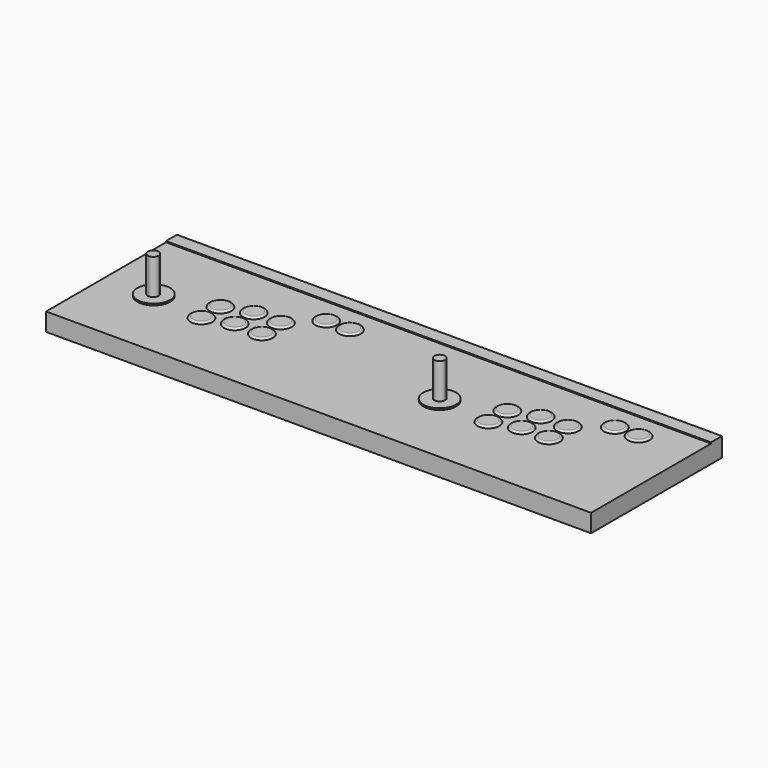
from build123d import *

# Parameters (mm, degrees)
F0_W     = 1000
F0_H     = 35
F1_DEPTH = 300
F2_W     = 1000
F2_H     = 275
F3_DEPTH = 2
F4_R     = 30
F4_R_2   = 20
F5_DEPTH = 3
F8_DEPTH = 65


# Not quite as in the source:
# - a fillet or chamfer that OpenCascade refuses, or shapes differently, is made with other operations: its cross-section is extruded or revolved along the edge and cut away or added


with BuildPart() as f1:
    # F0 (on Front) → F1 (new body)
    with BuildSketch(Plane.XZ):
        with Locations((415.1359161552, 9.4094127417)):
            Rectangle(F0_W, F0_H)
    extrude(amount=F1_DEPTH)

    # F2 (on face) → F3 (cut)
    with BuildSketch(Plane.XY.offset(26.9094127417)):
        with Locations((415.1359161552, -162.5)):
            Rectangle(F2_W, F2_H)
    extrude(amount=-F3_DEPTH, mode=Mode.SUBTRACT)

    # F4 (on face) → F5 (join)
    with BuildSketch(Plane.XY.offset(24.9094127417)):
        with Locations((5.3150048805, -165.6954972839)):
            Circle(F4_R)
        with Locations((101.5675663948, -176.7151132226)):
            Circle(F4_R_2)
        with Locations((101.5675638381, -133.2076661438)):
            Circle(F4_R_2)
        with Locations((150.2870444718, -117.7002512067)):
            Circle(F4_R_2)
        with Locations((200.0602781773, -161.2076982856)):
            Circle(F4_R_2)
        with Locations((200.0602756206, -117.7002512067)):
            Circle(F4_R_2)
        with Locations((150.2870470285, -161.2076982856)):
            Circle(F4_R_2)
        with Locations((247.0354534834, -72.4265153941)):
            Circle(F4_R_2)
        with Locations((290.5429005623, -72.4265128374)):
            Circle(F4_R_2)
        with Locations((527.8573036194, -163.2558181882)):
            Circle(F4_R)
        with Locations((624.1627931595, -171.8313768506)):
            Circle(F4_R_2)
        with Locations((624.1627906028, -128.3239297718)):
            Circle(F4_R_2)
        with Locations((672.8822712365, -112.8165148347)):
            Circle(F4_R_2)
        with Locations((672.8822737932, -156.3239619136)):
            Circle(F4_R_2)
        with Locations((722.6555049419, -156.3239619136)):
            Circle(F4_R_2)
        with Locations((722.6555023852, -112.8165148347)):
            Circle(F4_R_2)
        with Locations((776.1480905264, -71.8160520729)):
            Circle(F4_R_2)
        with Locations((819.6555376053, -71.8160495162)):
            Circle(F4_R_2)
    extrude(amount=F5_DEPTH)

    # F6: fillet of radius 5 on 16 edges, made by hand

    # F6_s1 → F6_t2 (revolve, cut)
    with BuildSketch(Plane.XZ.offset(176.7151132226)):
        with BuildLine():
            ThreePointArc((121.5675663948, 24.9094127417), (119.7236034874, 27.0927128743), (116.9849906999, 27.9094127417))
            Line((116.9849906999, 27.9094127417), (121.5675663948, 27.9094127417))
            Line((121.5675663948, 27.9094127417), (121.5675663948, 24.9094127417))
        make_face()
    revolve(axis=Axis((101.5675663948, -176.7151132226, 27.9094127417), (0, 0, 1)), mode=Mode.SUBTRACT)

    # F6_s3 → F6_t4 (revolve, cut)
    with BuildSketch(Plane.XZ.offset(133.2076661438)):
        with BuildLine():
            ThreePointArc((121.5675638381, 24.9094127417), (119.7236009307, 27.0927128743), (116.9849881431, 27.9094127417))
            Line((116.9849881431, 27.9094127417), (121.5675638381, 27.9094127417))
            Line((121.5675638381, 27.9094127417), (121.5675638381, 24.9094127417))
        make_face()
    revolve(axis=Axis((101.5675638381, -133.2076661438, 27.9094127417), (0, 0, 1)), mode=Mode.SUBTRACT)

    # F6_s5 → F6_t6 (revolve, cut)
    with BuildSketch(Plane.XZ.offset(117.7002512067)):
        with BuildLine():
            ThreePointArc((170.2870444718, 24.9094127417), (168.4430815644, 27.0927128743), (165.7044687769, 27.9094127417))
            Line((165.7044687769, 27.9094127417), (170.2870444718, 27.9094127417))
            Line((170.2870444718, 27.9094127417), (170.2870444718, 24.9094127417))
        make_face()
    revolve(axis=Axis((150.2870444718, -117.7002512067, 27.9094127417), (0, 0, 1)), mode=Mode.SUBTRACT)

    # F6_s7 → F6_t8 (revolve, cut)
    with BuildSketch(Plane.XZ.offset(161.2076982856)):
        with BuildLine():
            ThreePointArc((170.2870470285, 24.9094127417), (168.4430841211, 27.0927128743), (165.7044713336, 27.9094127417))
            Line((165.7044713336, 27.9094127417), (170.2870470285, 27.9094127417))
            Line((170.2870470285, 27.9094127417), (170.2870470285, 24.9094127417))
        make_face()
    revolve(axis=Axis((150.2870470285, -161.2076982856, 27.9094127417), (0, 0, 1)), mode=Mode.SUBTRACT)

    # F6_s9 → F6_t10 (revolve, cut)
    with BuildSketch(Plane.XZ.offset(161.2076982856)):
        with BuildLine():
            ThreePointArc((220.0602781773, 24.9094127417), (218.2163152698, 27.0927128743), (215.4777024823, 27.9094127417))
            Line((215.4777024823, 27.9094127417), (220.0602781773, 27.9094127417))
            Line((220.0602781773, 27.9094127417), (220.0602781773, 24.9094127417))
        make_face()
    revolve(axis=Axis((200.0602781773, -161.2076982856, 27.9094127417), (0, 0, 1)), mode=Mode.SUBTRACT)

    # F6_s11 → F6_t12 (revolve, cut)
    with BuildSketch(Plane.XZ.offset(117.7002512067)):
        with BuildLine():
            ThreePointArc((220.0602756206, 24.9094127417), (218.2163127131, 27.0927128743), (215.4776999256, 27.9094127417))
            Line((215.4776999256, 27.9094127417), (220.0602756206, 27.9094127417))
            Line((220.0602756206, 27.9094127417), (220.0602756206, 24.9094127417))
        make_face()
    revolve(axis=Axis((200.0602756206, -117.7002512067, 27.9094127417), (0, 0, 1)), mode=Mode.SUBTRACT)

    # F6_s13 → F6_t14 (revolve, cut)
    with BuildSketch(Plane.XZ.offset(72.4265153941)):
        with BuildLine():
            ThreePointArc((267.0354534834, 24.9094127417), (265.191490576, 27.0927128743), (262.4528777885, 27.9094127417))
            Line((262.4528777885, 27.9094127417), (267.0354534834, 27.9094127417))
            Line((267.0354534834, 27.9094127417), (267.0354534834, 24.9094127417))
        make_face()
    revolve(axis=Axis((247.0354534834, -72.4265153941, 27.9094127417), (0, 0, 1)), mode=Mode.SUBTRACT)

    # F6_s15 → F6_t16 (revolve, cut)
    with BuildSketch(Plane.XZ.offset(72.4265128374)):
        with BuildLine():
            ThreePointArc((310.5429005623, 24.9094127417), (308.6989376549, 27.0927128743), (305.9603248673, 27.9094127417))
            Line((305.9603248673, 27.9094127417), (310.5429005623, 27.9094127417))
            Line((310.5429005623, 27.9094127417), (310.5429005623, 24.9094127417))
        make_face()
    revolve(axis=Axis((290.5429005623, -72.4265128374, 27.9094127417), (0, 0, 1)), mode=Mode.SUBTRACT)

    # F6_s17 → F6_t18 (revolve, cut)
    with BuildSketch(Plane.XZ.offset(71.8160495162)):
        with BuildLine():
            ThreePointArc((839.6555376053, 24.9094127417), (837.8115746979, 27.0927128743), (835.0729619103, 27.9094127417))
            Line((835.0729619103, 27.9094127417), (839.6555376053, 27.9094127417))
            Line((839.6555376053, 27.9094127417), (839.6555376053, 24.9094127417))
        make_face()
    revolve(axis=Axis((819.6555376053, -71.8160495162, 27.9094127417), (0, 0, 1)), mode=Mode.SUBTRACT)

    # F6_s19 → F6_t20 (revolve, cut)
    with BuildSketch(Plane.XZ.offset(71.8160520729)):
        with BuildLine():
            ThreePointArc((796.1480905264, 24.9094127417), (794.304127619, 27.0927128743), (791.5655148315, 27.9094127417))
            Line((791.5655148315, 27.9094127417), (796.1480905264, 27.9094127417))
            Line((796.1480905264, 27.9094127417), (796.1480905264, 24.9094127417))
        make_face()
    revolve(axis=Axis((776.1480905264, -71.8160520729, 27.9094127417), (0, 0, 1)), mode=Mode.SUBTRACT)

    # F6_s21 → F6_t22 (revolve, cut)
    with BuildSketch(Plane.XZ.offset(112.8165148347)):
        with BuildLine():
            ThreePointArc((742.6555023852, 24.9094127417), (740.8115394778, 27.0927128743), (738.0729266903, 27.9094127417))
            Line((738.0729266903, 27.9094127417), (742.6555023852, 27.9094127417))
            Line((742.6555023852, 27.9094127417), (742.6555023852, 24.9094127417))
        make_face()
    revolve(axis=Axis((722.6555023852, -112.8165148347, 27.9094127417), (0, 0, 1)), mode=Mode.SUBTRACT)

    # F6_s23 → F6_t24 (revolve, cut)
    with BuildSketch(Plane.XZ.offset(156.3239619136)):
        with BuildLine():
            ThreePointArc((742.6555049419, 24.9094127417), (740.8115420345, 27.0927128743), (738.072929247, 27.9094127417))
            Line((738.072929247, 27.9094127417), (742.6555049419, 27.9094127417))
            Line((742.6555049419, 27.9094127417), (742.6555049419, 24.9094127417))
        make_face()
    revolve(axis=Axis((722.6555049419, -156.3239619136, 27.9094127417), (0, 0, 1)), mode=Mode.SUBTRACT)

    # F6_s25 → F6_t26 (revolve, cut)
    with BuildSketch(Plane.XZ.offset(156.3239619136)):
        with BuildLine():
            ThreePointArc((692.8822737932, 24.9094127417), (691.0383108858, 27.0927128743), (688.2996980983, 27.9094127417))
            Line((688.2996980983, 27.9094127417), (692.8822737932, 27.9094127417))
            Line((692.8822737932, 27.9094127417), (692.8822737932, 24.9094127417))
        make_face()
    revolve(axis=Axis((672.8822737932, -156.3239619136, 27.9094127417), (0, 0, 1)), mode=Mode.SUBTRACT)

    # F6_s27 → F6_t28 (revolve, cut)
    with BuildSketch(Plane.XZ.offset(112.8165148347)):
        with BuildLine():
            ThreePointArc((692.8822712365, 24.9094127417), (691.0383083291, 27.0927128743), (688.2996955416, 27.9094127417))
            Line((688.2996955416, 27.9094127417), (692.8822712365, 27.9094127417))
            Line((692.8822712365, 27.9094127417), (692.8822712365, 24.9094127417))
        make_face()
    revolve(axis=Axis((672.8822712365, -112.8165148347, 27.9094127417), (0, 0, 1)), mode=Mode.SUBTRACT)

    # F6_s29 → F6_t30 (revolve, cut)
    with BuildSketch(Plane.XZ.offset(128.3239297718)):
        with BuildLine():
            ThreePointArc((644.1627906028, 24.9094127417), (642.3188276953, 27.0927128743), (639.5802149078, 27.9094127417))
            Line((639.5802149078, 27.9094127417), (644.1627906028, 27.9094127417))
            Line((644.1627906028, 27.9094127417), (644.1627906028, 24.9094127417))
        make_face()
    revolve(axis=Axis((624.1627906028, -128.3239297718, 27.9094127417), (0, 0, 1)), mode=Mode.SUBTRACT)

    # F6_s31 → F6_t32 (revolve, cut)
    with BuildSketch(Plane.XZ.offset(171.8313768506)):
        with BuildLine():
            ThreePointArc((644.1627931595, 24.9094127417), (642.3188302521, 27.0927128743), (639.5802174645, 27.9094127417))
            Line((639.5802174645, 27.9094127417), (644.1627931595, 27.9094127417))
            Line((644.1627931595, 27.9094127417), (644.1627931595, 24.9094127417))
        make_face()
    revolve(axis=Axis((624.1627931595, -171.8313768506, 27.9094127417), (0, 0, 1)), mode=Mode.SUBTRACT)

    # F7 (on face) → F8 (join)
    with BuildSketch(Plane.XY.offset(27.9094127417)):
        with BuildLine():
            ThreePointArc((4.4260412971, -175.935565011), (11.497109109, -173.0066328229), (14.4260412971, -165.935565011))
            Line((14.4260412971, -165.935565011), (4.4260412971, -165.935565011))
            Line((4.4260412971, -165.935565011), (4.4260412971, -175.935565011))
        make_face()
        with BuildLine():
            Line((4.4260412971, -175.935565011), (4.4260412971, -165.935565011))
            Line((4.4260412971, -165.935565011), (-5.5739587029, -165.935565011))
            ThreePointArc((-5.5739587029, -165.935565011), (-2.6450265147, -173.0066328229), (4.4260412971, -175.935565011))
        make_face()
        with BuildLine():
            Line((-5.5739587029, -165.935565011), (4.4260412971, -165.935565011))
            Line((4.4260412971, -165.935565011), (4.4260412971, -155.935565011))
            ThreePointArc((4.4260412971, -155.935565011), (-2.6450265147, -158.8644971991), (-5.5739587029, -165.935565011))
        make_face()
        with BuildLine():
            Line((4.4260412971, -165.935565011), (14.4260412971, -165.935565011))
            ThreePointArc((14.4260412971, -165.935565011), (11.497109109, -158.8644971991), (4.4260412971, -155.935565011))
            Line((4.4260412971, -155.935565011), (4.4260412971, -165.935565011))
        make_face()
        with BuildLine():
            Line((537.2473394871, -162.224188447), (526.3316631317, -162.224188447))
            Line((526.3316631317, -162.224188447), (526.3316631317, -172.1821770397))
            ThreePointArc((526.3316631317, -172.1821770397), (533.9868957205, -169.6119067535), (537.2473394871, -162.224188447))
        make_face()
        with BuildLine():
            Line((526.3316631317, -172.1821770397), (526.3316631317, -162.224188447))
            Line((526.3316631317, -162.224188447), (517.2473394871, -162.224188447))
            ThreePointArc((517.2473394871, -162.224188447), (519.8596211805, -168.9637446804), (526.3316631317, -172.1821770397))
        make_face()
        with BuildLine():
            Line((526.3316631317, -162.224188447), (526.3316631317, -152.2661998543))
            ThreePointArc((526.3316631317, -152.2661998543), (519.8596211805, -155.4846322136), (517.2473394871, -162.224188447))
            Line((517.2473394871, -162.224188447), (526.3316631317, -162.224188447))
        make_face()
        with BuildLine():
            ThreePointArc((537.2473394871, -162.224188447), (533.9868957205, -154.8364701405), (526.3316631317, -152.2661998543))
            Line((526.3316631317, -152.2661998543), (526.3316631317, -162.224188447))
            Line((526.3316631317, -162.224188447), (537.2473394871, -162.224188447))
        make_face()
    extrude(amount=F8_DEPTH)


solid = f1.part
